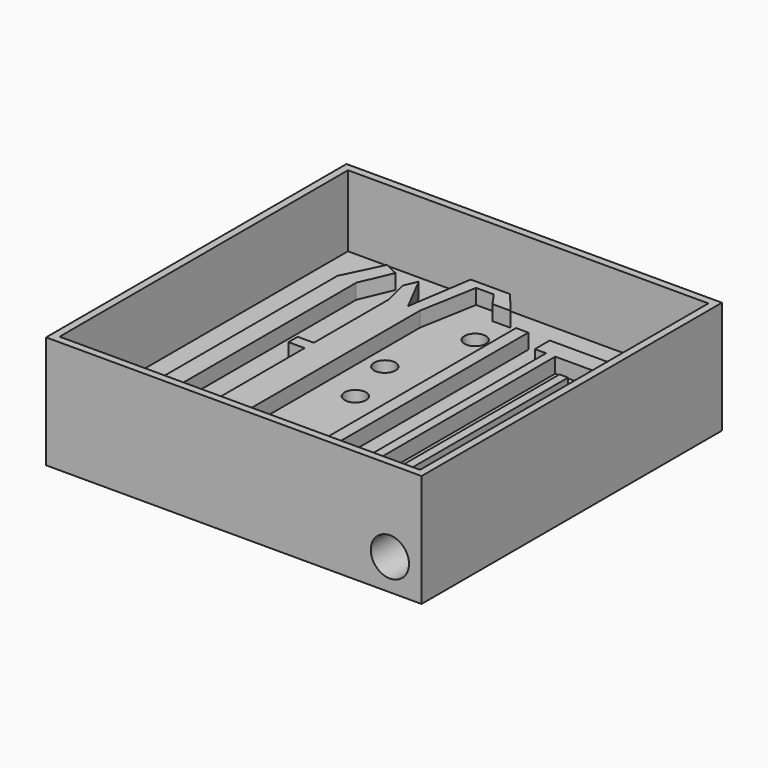
from build123d import *

# Parameters (mm, degrees)
F0_W          = 100
F0_H          = 100
F1_DEPTH      = 30
F2_W          = 96
F2_H          = 96
F3_DEPTH      = 15
F4_R          = 2.85
F4_R_2        = 3.6776726438
F5_DEPTH      = 4
F6_DEPTH      = 7.5
F5_FACE_R     = 2.85
F7_DEPTH      = 7.5
F8_DEPTH      = 7.5
F9_DEPTH      = 7.5
F10_R         = 5.0877559258
F11_DEPTH     = 11
F12_TEXT_SIZE = 4.6145616633
F13_DEPTH     = 2
F14_R         = 2.85
F15_DEPTH     = 1
F16_TEXT_SIZE = 1.6368201209
F17_DEPTH     = 1


# Not quite as in the source:
# - Text() gives the source's letters only with a copy of the font that has no kerning and outlines rounded to 1/6400 em; it was checked with that copy


with BuildPart() as f1:
    # F0 (on Top) → F1 (new body)
    with BuildSketch(Plane.XY):
        Rectangle(F0_W, F0_H)
    extrude(amount=F1_DEPTH)

    # F2 (on face) → F3 (cut)
    with BuildSketch(Plane.XY.offset(30)):
        Rectangle(F2_W, F2_H)
    extrude(amount=-F3_DEPTH, mode=Mode.SUBTRACT)

    # F4 (on face) → F5 (cut)
    with BuildSketch(Plane.XY.offset(15)):
        Polygon((-48, -48), (-38, -48), (-38, 32), (-33, 42.3), (-29.3782448554, 40.5418664346), (-33, 32), (-33, -48), (5.7, -48), (5.7, 36.8372872472), (8.9758234099, 36.8372872472), (8.9758234099, -48), (25.8013814658, -48), (25.8013814658, 26.180415976), (28.0806608498, 26.180415976), (28.0806608498, -39.1144752502), (37.0941460133, -39.1144752502), (37.0941460133, -42.3), (28.0806608498, -42.3), (28.0806608498, -48), (48, -48), (48, -33.4144752502), (33.7806608498, -33.4144752502), (33.7806608498, -25.1540765166), (48, -25.1540765166), (48, 9.7570158541), (33.7806608498, 9.7570158541), (33.7806608498, 17.218105495), (48, 17.218105495), (48, 31.880415976), (23.2517495751, 31.880415976), (20.1013814658, 31.880415976), (20.1013814658, -42.3), (17.6548361778, -42.3), (17.6548361778, 31.880415976), (14.6758234099, 31.880415976), (14.6758234099, 36.8372872472), (23.2517495751, 36.8372872472), (48, 36.8372872472), (48, 48), (-4.8668491654, 48), (0, 42.1958640218), (-4.8668491654, 42.1958640218), (-7.3829777539, 45.7755178213), (-12.0867760852, 45.7755178213), (-14.8065052927, 30.4983254224), (-14.8065052927, -37.2936502099), (-12.0867760852, -37.2936502099), (0, -37.2936502099), (0, -40.2936502099), (-14.8065052927, -40.2936502099), (-18, -40.2936502099), (-18, -43), (-23, -43), (-23, 2.3087414447), (-27.3, 2.3087414447), (-27.3, 5.3887376562), (-23, 5.3887376562), (-23, 30.4983254224), (-24.649743792, 37.0921127731), (-23.1870467144, 40.5418664346), (-18, 30.4983254224), (-15.3014808893, 48), (-48, 48), align=None)
        with Locations((-6.0123181902, -2.0270207897)):
            Circle(F4_R, mode=Mode.SUBTRACT)
        with Locations((0, -27.3110400885)):
            Circle(F4_R, mode=Mode.SUBTRACT)
        with Locations((41.8636836112, -43.1411899626)):
            Circle(F4_R_2, mode=Mode.SUBTRACT)
        with Locations((-9.5676705241, 12.2440252453)):
            Circle(F4_R, mode=Mode.SUBTRACT)
        with Locations((-2.4050001521, 33.3630181849)):
            Circle(F4_R, mode=Mode.SUBTRACT)
    extrude(amount=-F5_DEPTH, mode=Mode.SUBTRACT)

    # F6 (cut): a face of the model
    f6_faces = [f1.faces().sort_by_distance(p)[0] for p in [
        (41.8636836112, -43.1411899626, 15),
    ]]
    extrude(f6_faces, amount=-F6_DEPTH, mode=Mode.SUBTRACT)

    # F2 (on face) + F5_face (on face) → F7 (cut)
    with BuildSketch(Plane.XY.offset(30)):
        Rectangle(F2_W, F2_H)
    with BuildSketch(Plane(origin=(41.8636836112, -43.1411899626, 15), x_dir=(1, 0, 0), z_dir=(0, 0, 1))):
        with Locations((-44.2686837632, 76.5042081475)):
            Circle(F5_FACE_R)
    extrude(amount=-F7_DEPTH, mode=Mode.SUBTRACT)

    # F8 (cut): a face of the model
    f8_faces = [f1.faces().sort_by_distance(p)[0] for p in [
        (-9.5676705241, 12.2440252453, 15),
    ]]
    extrude(f8_faces, amount=-F8_DEPTH, mode=Mode.SUBTRACT)

    # F9 (cut): faces of the model
    f9_faces = [f1.faces().sort_by_distance(p)[0] for p in [
        (-6.0123181902, -2.0270207897, 15),
        (0, -27.3110400885, 15),
    ]]
    extrude(f9_faces, amount=-F9_DEPTH, mode=Mode.SUBTRACT)

    # F10 (on face) → F11 (cut)
    with BuildSketch(Plane.XZ.offset(50)):
        with Locations((41.5709763765, 8.3122440742)):
            Circle(F10_R)
    extrude(amount=-F11_DEPTH, mode=Mode.SUBTRACT)

    # F12 (on face) → F13 (cut)
    with BuildSketch(Plane.XY.offset(15)):
        with Locations((33.7806608498, -30.4765609142)):
            Text('FINISH', F12_TEXT_SIZE, font='Open Sans', text_align=(TextAlign.LEFT, TextAlign.BOTTOM))
    extrude(amount=-F13_DEPTH, mode=Mode.SUBTRACT)

    # F14 (on face) → F15 (cut)
    with BuildSketch(Plane.XY.offset(11)):
        with Locations((-43.5000546277, -44.8192730546)):
            Circle(F14_R)
    extrude(amount=-F15_DEPTH, mode=Mode.SUBTRACT)

    # F16 (on face) → F17 (join)
    with BuildSketch(Plane.XY.offset(11)):
        with Locations((-45.249287039, -40.1654131711)):
            Text('Start', F16_TEXT_SIZE, font='Open Sans', text_align=(TextAlign.LEFT, TextAlign.BOTTOM))
    extrude(amount=F17_DEPTH)


solid = f1.part
